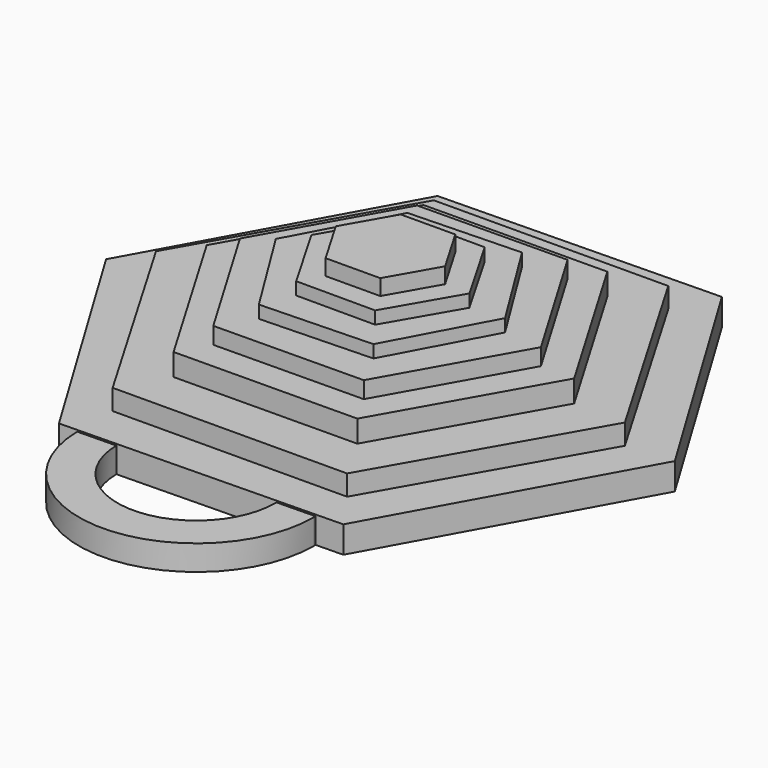
from build123d import *

# Parameters (mm, degrees)
F1_DEPTH      = 4.318
F3_DEPTH      = 3.302
F5_DEPTH      = 3.556
F7_DEPTH      = 2.6924
F9_DEPTH      = 2.032
F11_DEPTH     = 2.032
F13_DEPTH     = 2.54
F14_TEXT_SIZE = 45.3219283372
F15_DEPTH     = 1.524
F17_DEPTH     = 4.064


# Not quite as in the source:
# - Text() gives the source's letters only with a copy of the font that has no kerning and outlines rounded to 1/6400 em; it was checked with that copy


with BuildPart() as f1:
    # F0 (on Top) → F1 (new body)
    with BuildSketch(Plane.XY):
        Polygon((23.3215753213, -38.6437264325), (45.1272364481, 0.8752134683), (21.8056611268, 39.5189399008), (-23.3215753213, 38.6437264325), (-45.1272364481, -0.8752134683), (-21.8056611268, -39.5189399008), align=None)
    extrude(amount=F1_DEPTH)

    # F2 (on face) → F3 (join)
    with BuildSketch(Plane.XY.offset(4.318)):
        Polygon((18.9851936436, -32.4725893565), (37.6146841311, 0.2053653129), (18.6294904876, 32.6779546693), (-18.9851936436, 32.4725893565), (-37.6146841311, -0.2053653129), (-18.6294904876, -32.6779546693), align=None)
    extrude(amount=F3_DEPTH)

    # F4 (on face) → F5 (join)
    with BuildSketch(Plane.XY.offset(7.62)):
        Polygon((14.9258637315, -25.3329233865), (29.4018870706, 0.2597154716), (14.4760233391, 25.5926388581), (-14.9258637315, 25.3329233865), (-29.4018870706, -0.2597154716), (-14.4760233391, -25.5926388581), align=None)
    extrude(amount=F5_DEPTH)

    # F6 (on face) → F7 (join)
    with BuildSketch(Plane.XY.offset(11.176)):
        Polygon((12.2494456955, -20.6844104103), (24.0379477254, 0.2661259494), (11.7885020299, 20.9505363598), (-12.2494456955, 20.6844104103), (-24.0379477254, -0.2661259494), (-11.7885020299, -20.9505363598), align=None)
    extrude(amount=F7_DEPTH)

    # F8 (on face) → F9 (join)
    with BuildSketch(Plane.XY.offset(13.8684)):
        Polygon((9.5047761585, -15.3033065358), (18.0054403012, 0.5797243426), (8.5006641427, 15.8830308784), (-9.5047761585, 15.3033065358), (-18.0054403012, -0.5797243426), (-8.5006641427, -15.8830308784), align=None)
    extrude(amount=F9_DEPTH)

    # F10 (on face) → F11 (join)
    with BuildSketch(Plane.XY.offset(15.9004)):
        Polygon((6.3575136843, -11.0353062281), (12.7356123742, -0.0118847585), (6.3780986899, 11.0234214696), (-6.3575136843, 11.0353062281), (-12.7356123742, 0.0118847585), (-6.3780986899, -11.0234214696), align=None)
    extrude(amount=F11_DEPTH)

    # F12 (on face) → F13 (join)
    with BuildSketch(Plane.XY.offset(17.9324)):
        Polygon((4.427027495, -7.5797649104), (8.7777827146, 0.0440358187), (4.3507552196, 7.6238007291), (-4.427027495, 7.5797649104), (-8.7777827146, -0.0440358187), (-4.3507552196, -7.6238007291), align=None)
    extrude(amount=F13_DEPTH)

    # F14 (on face) → F15 (cut)
    with BuildSketch(Plane(origin=(0, 0, 0), x_dir=(1, 0, 0), z_dir=(0, 0, -1))):
        with Locations((-26.7207363504, -14.4146803614)):
            Text('RP', F14_TEXT_SIZE, font='Open Sans', font_style=FontStyle.BOLDITALIC, text_align=(TextAlign.LEFT, TextAlign.BOTTOM))
    extrude(amount=-F15_DEPTH, mode=Mode.SUBTRACT)

    # F16 (on face) → F17 (join)
    with BuildSketch(Plane(origin=(0, 0, 0), x_dir=(1, 0, 0), z_dir=(0, 0, -1))):
        with BuildLine():
            ThreePointArc((18.9180054607, 38.7291308125), (18.9206736269, 38.912573409), (18.9215630435, 39.0960332527))
            ThreePointArc((18.9215630435, 39.0960332527), (0.1834598437, 58.0167068797), (-18.9180054607, 39.4629356929))
            Line((-18.9180054607, 39.4629356929), (-12.7045055264, 39.3424288936))
            ThreePointArc((-12.7045055264, 39.3424288936), (0.1232036117, 51.802330603), (12.7068946436, 39.0960332527))
            ThreePointArc((12.7068946436, 39.0960332527), (12.7062973502, 38.9728296411), (12.7045055264, 38.8496376119))
            Line((12.7045055264, 38.8496376119), (18.9180054607, 38.7291308125))
        make_face()
    extrude(amount=-F17_DEPTH)


solid = f1.part
